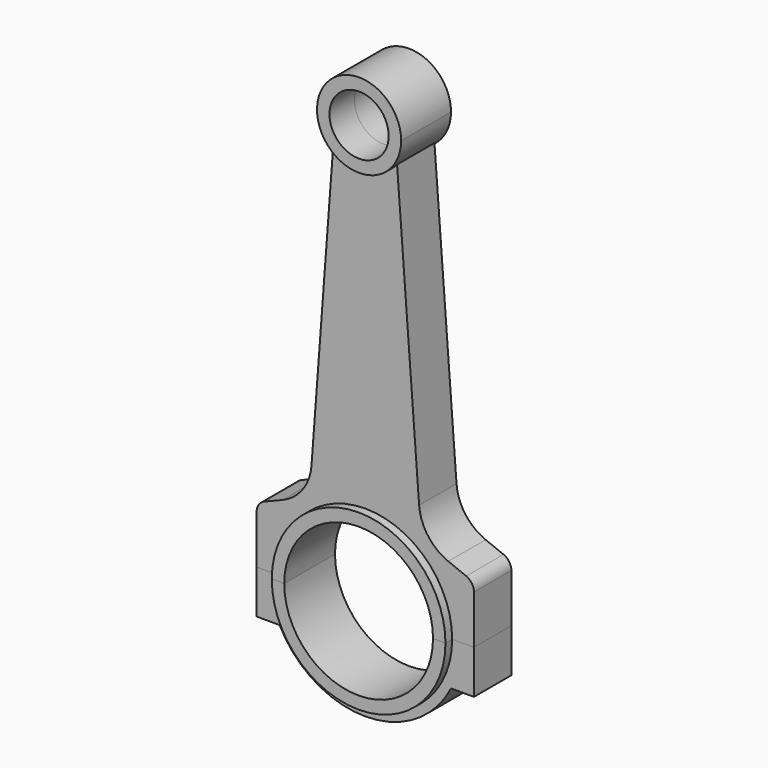
from build123d import *

# Parameters (mm, degrees)
F1_DEPTH = 12.9286
F2_DEPTH = 9.525
F3_DEPTH = 12.9286
F4_DEPTH = 9.525
F0_R     = 12.065
F5_DEPTH = 12.7


with BuildPart() as f1:
    # F0 (on Front) → F1 (new body, symmetric)
    with BuildSketch(Plane.XZ):
        with BuildLine():
            ThreePointArc((-30.3149, -69.2796702024), (0, -38.9647702024), (30.3149, -69.2796702024))
            Line((30.3149, -69.2796702024), (35.3949, -69.2796702024))
            ThreePointArc((35.3949, -69.2796702024), (0, -33.8847702024), (-35.3949, -69.2796702024))
            Line((-35.3949, -69.2796702024), (-30.3149, -69.2796702024))
        make_face()
    extrude(amount=F1_DEPTH, both=True)

    # F0 (on Front) → F2 (join, symmetric)
    with BuildSketch(Plane.XZ):
        with BuildLine():
            ThreePointArc((-39.2049, -69.2796702024), (0, -30.0747702024), (39.2049, -69.2796702024))
            Line((39.2049, -69.2796702024), (44.2849, -69.2796702024))
            Line((44.2849, -69.2796702024), (44.2849, -49.4660918501))
            ThreePointArc((44.2849, -49.4660918501), (43.4141556404, -46.6220512467), (41.1004248213, -44.7529839952))
            Line((41.1004248213, -44.7529839952), (33.8186777373, -41.8243999769))
            ThreePointArc((33.8186777373, -41.8243999769), (25.5540866411, -35.4009894091), (21.9306908548, -25.5808737129))
            Line((21.9306908548, -25.5808737129), (12.9457367136, 93.7233811748))
            ThreePointArc((12.9457367136, 93.7233811748), (0, 87.8193297976), (-12.9457367136, 93.7233811748))
            Line((-12.9457367136, 93.7233811748), (-21.9306908548, -25.5808737129))
            ThreePointArc((-21.9306908548, -25.5808737129), (-25.5540866411, -35.4009894091), (-33.8186777373, -41.8243999769))
            Line((-33.8186777373, -41.8243999769), (-41.1004248213, -44.7529839952))
            ThreePointArc((-41.1004248213, -44.7529839952), (-43.4141556404, -46.6220512467), (-44.2849, -49.4660918501))
            Line((-44.2849, -49.4660918501), (-44.2849, -69.2796702024))
            Line((-44.2849, -69.2796702024), (-39.2049, -69.2796702024))
        make_face()
        with BuildLine():
            ThreePointArc((-35.3949, -69.2796702024), (0, -33.8847702024), (35.3949, -69.2796702024))
            Line((35.3949, -69.2796702024), (39.2049, -69.2796702024))
            ThreePointArc((39.2049, -69.2796702024), (0, -30.0747702024), (-39.2049, -69.2796702024))
            Line((-39.2049, -69.2796702024), (-35.3949, -69.2796702024))
        make_face()
    extrude(amount=F2_DEPTH, both=True)

    # F0 (on Front) → F5 (join, symmetric)
    with BuildSketch(Plane.XZ):
        with BuildLine():
            ThreePointArc((-12.9457367136, 93.7233811748), (0, 87.8193297976), (12.9457367136, 93.7233811748))
            ThreePointArc((12.9457367136, 93.7233811748), (16.0609103253, 98.9644810893), (17.145, 104.9643297976))
            ThreePointArc((17.145, 104.9643297976), (-5.9998487083, 121.0252401229), (-12.9457367136, 93.7233811748))
        make_face()
        with Locations((0, 104.9643297976)):
            Circle(F0_R, mode=Mode.SUBTRACT)
    extrude(amount=F5_DEPTH, both=True)


with BuildPart() as f3:
    # F0 (on Front) → F3 (new body, symmetric)
    with BuildSketch(Plane.XZ):
        with BuildLine():
            Line((35.3949, -69.2796702024), (30.3149, -69.2796702024))
            ThreePointArc((30.3149, -69.2796702024), (0, -99.5945702024), (-30.3149, -69.2796702024))
            Line((-30.3149, -69.2796702024), (-35.3949, -69.2796702024))
            ThreePointArc((-35.3949, -69.2796702024), (0, -104.6745702024), (35.3949, -69.2796702024))
        make_face()
    extrude(amount=F3_DEPTH, both=True)

    # F0 (on Front) → F4 (join, symmetric)
    with BuildSketch(Plane.XZ):
        with BuildLine():
            ThreePointArc((-34.941319151, -87.0596702024), (-38.1241072498, -78.4216957117), (-39.2049, -69.2796702024))
            Line((-39.2049, -69.2796702024), (-44.2849, -69.2796702024))
            Line((-44.2849, -69.2796702024), (-44.2849, -87.0596702024))
            Line((-44.2849, -87.0596702024), (-34.941319151, -87.0596702024))
        make_face()
        with BuildLine():
            Line((39.2049, -69.2796702024), (35.3949, -69.2796702024))
            ThreePointArc((35.3949, -69.2796702024), (0, -104.6745702024), (-35.3949, -69.2796702024))
            Line((-35.3949, -69.2796702024), (-39.2049, -69.2796702024))
            ThreePointArc((-39.2049, -69.2796702024), (-38.1241072498, -78.4216957117), (-34.941319151, -87.0596702024))
            ThreePointArc((-34.941319151, -87.0596702024), (0, -108.4845702024), (34.941319151, -87.0596702024))
            ThreePointArc((34.941319151, -87.0596702024), (38.1241072498, -78.4216957117), (39.2049, -69.2796702024))
        make_face()
        with BuildLine():
            Line((44.2849, -69.2796702024), (39.2049, -69.2796702024))
            ThreePointArc((39.2049, -69.2796702024), (38.1241072498, -78.4216957117), (34.941319151, -87.0596702024))
            Line((34.941319151, -87.0596702024), (44.2849, -87.0596702024))
            Line((44.2849, -87.0596702024), (44.2849, -69.2796702024))
        make_face()
    extrude(amount=F4_DEPTH, both=True)


solid = Compound([f1.part, f3.part])
